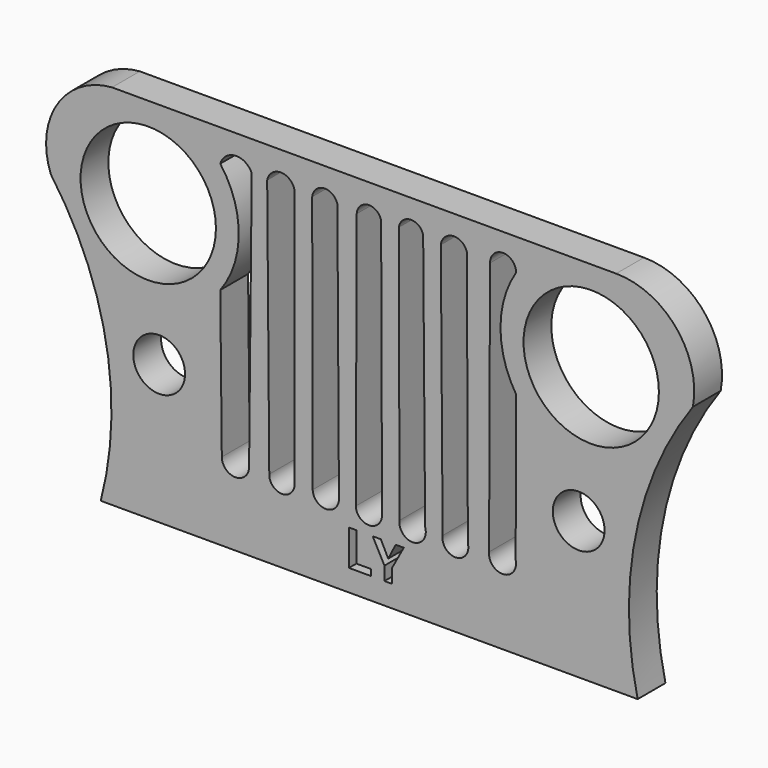
from build123d import *

# Parameters (mm, degrees)
F0_R         = 3.725
F0_R_2       = 9.74
F1_DEPTH     = 5
F2_TEXT_SIZE = 7.1775700935
F3_DEPTH     = 25


# Not quite as in the source:
# - Text() gives the source's letters only with a copy of the font that has no kerning and outlines rounded to 1/6400 em; it was checked with that copy


with BuildPart() as f1:
    # F0 (on Front) → F1 (new body)
    with BuildSketch(Plane.XZ):
        with BuildLine():
            Line((34.936432234, 22.5417102225), (-37.6104430905, 22.5417102225))
            ThreePointArc((-37.6104430905, 22.5417102225), (-45.5115799605, 17.819386847), (-46.4175735166, 8.6592843597))
            ThreePointArc((-46.4175735166, 8.6592843597), (-38.4619662035, -10.048790614), (-39.2361740253, -30.363424728))
            Line((-39.2361740253, -30.363424728), (38.0289382026, -30.363424728))
            ThreePointArc((38.0289382026, -30.363424728), (37.7295941582, -9.6950682132), (45.9826696144, 9.2563779953))
            ThreePointArc((45.9826696144, 9.2563779953), (43.5752894016, 18.4896595522), (34.936432234, 22.5417102225))
        make_face()
        with Locations((-30.8308005333, -10.3563340381)):
            Circle(F0_R, mode=Mode.SUBTRACT)
        with Locations((29.543550685, -10.5398427695)):
            Circle(F0_R, mode=Mode.SUBTRACT)
        with BuildLine():
            ThreePointArc((-22.0362562686, 17.9410949349), (-19.8711330315, 19.6582266779), (-17.5069794059, 18.2274654508))
            Line((-17.5069794059, 18.2274654508), (-17.8896225989, -19.1456079483))
            ThreePointArc((-17.8896225989, -19.1456079483), (-19.8515094817, -21.0853390303), (-21.8133963645, -19.1456079483))
            Line((-21.8133963645, -19.1456079483), (-22.0362562686, 1.935047796))
            ThreePointArc((-22.0362562686, 1.935047796), (-19.3728036853, 9.9380713655), (-22.0362562686, 17.9410949349))
        make_face(mode=Mode.SUBTRACT)
        with BuildLine():
            ThreePointArc((-15.2845885605, 18.0446933955), (-13.3181386627, 19.6676491024), (-11.351688765, 18.0446933955))
            Line((-11.351688765, 18.0446933955), (-11.3499974832, -18.9518425614))
            ThreePointArc((-11.3499974832, -18.9518425614), (-13.0874383842, -21.0025605146), (-14.983122237, -19.0971661359))
            Line((-14.983122237, -19.0971661359), (-15.2845885605, 18.0446933955))
        make_face(mode=Mode.SUBTRACT)
        with BuildLine():
            ThreePointArc((-2.396778902, 17.9841872305), (-0.7725597376, 19.6487813496), (1.1125782039, 18.2867180556))
            Line((1.1125782039, 18.2867180556), (1.244835672, -18.9518425614))
            ThreePointArc((1.244835672, -18.9518425614), (-0.5719654036, -20.9075458621), (-2.5336144026, -19.0971661359))
            Line((-2.5336144026, -19.0971661359), (-2.396778902, 17.9841872305))
        make_face(mode=Mode.SUBTRACT)
        with BuildLine():
            ThreePointArc((-8.8104307652, 18.0446933955), (-7.096420966, 19.6833293138), (-5.1800613292, 18.2867180556))
            Line((-5.1800613292, 18.2867180556), (-4.955697339, -18.903400749))
            ThreePointArc((-4.955697339, -18.903400749), (-6.7722604144, -20.8652873989), (-8.7341470644, -19.0487243235))
            Line((-8.7341470644, -19.0487243235), (-8.8104307652, 18.0446933955))
        make_face(mode=Mode.SUBTRACT)
        with Locations((-32.4004238579, 9.5442074278)):
            Circle(F0_R_2, mode=Mode.SUBTRACT)
        with BuildLine():
            ThreePointArc((3.6538355052, 18.2262118906), (5.333653558, 19.7642692571), (7.1631921455, 18.4077303857))
            Line((7.1631921455, 18.4077303857), (7.4453693815, -18.5158662498))
            ThreePointArc((7.4453693815, -18.5158662498), (5.8184140834, -21.0069679369), (3.7638025824, -18.8549589366))
            Line((3.7638025824, -18.8549589366), (3.6538355052, 18.2262118906))
        make_face(mode=Mode.SUBTRACT)
        with BuildLine():
            ThreePointArc((9.7044501454, 17.9841872305), (11.4559773654, 19.6750787949), (13.4558314458, 18.2867180556))
            Line((13.4558314458, 18.2867180556), (13.597461395, -18.5643080622))
            ThreePointArc((13.597461395, -18.5643080622), (11.9015951081, -20.9242457257), (9.9643357098, -18.7580753118))
            Line((9.9643357098, -18.7580753118), (9.7044501454, 17.9841872305))
        make_face(mode=Mode.SUBTRACT)
        with BuildLine():
            ThreePointArc((16.783669591, 17.9841872305), (18.6593607068, 19.8728887646), (20.5350518227, 17.9841872305))
            ThreePointArc((20.5350518227, 17.9841872305), (18.2896412527, 10.2681802819), (20.5350518227, 2.5521733332))
            Line((20.5350518227, 2.5521733332), (20.4761773348, -18.4189844877))
            ThreePointArc((20.4761773348, -18.4189844877), (18.7074826076, -20.8271691339), (16.6492853314, -18.661191687))
            Line((16.6492853314, -18.661191687), (16.783669591, 17.9841872305))
        make_face(mode=Mode.SUBTRACT)
        with Locations((31.3455425203, 9.5439981669)):
            Circle(F0_R_2, mode=Mode.SUBTRACT)
    extrude(amount=F1_DEPTH)

    # F2 (on face) → F3 (cut)
    with BuildSketch(Plane.XZ.offset(5)):
        with Locations((-4.1597038841, -27.2499331166)):
            Text('LY', F2_TEXT_SIZE, font='Open Sans', font_style=FontStyle.BOLD, text_align=(TextAlign.LEFT, TextAlign.BOTTOM))
    extrude(amount=-F3_DEPTH, mode=Mode.SUBTRACT)


solid = f1.part
